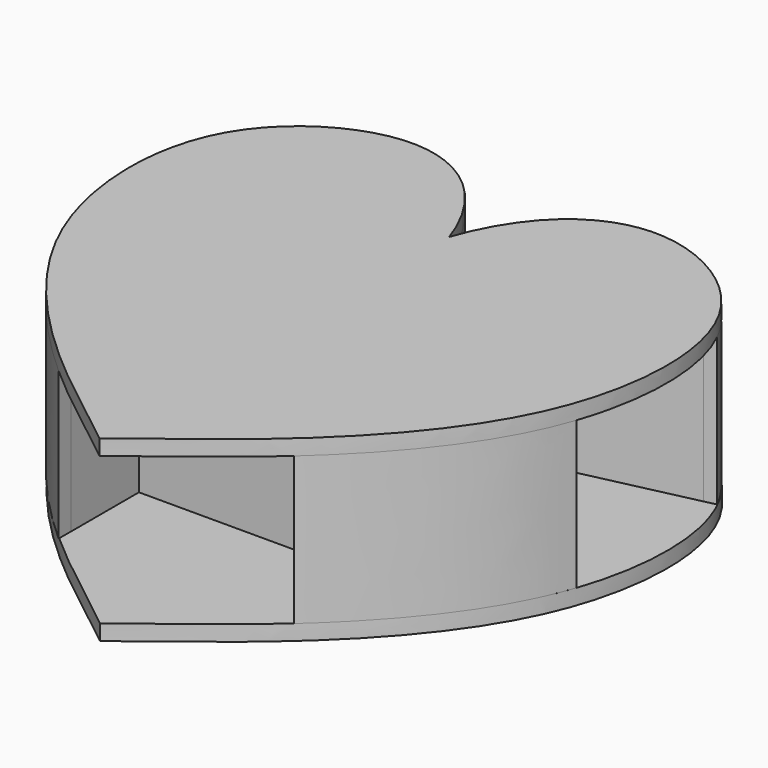
from build123d import *

# Parameters (mm, degrees)
F2_DEPTH = 4
F3_DEPTH = 38
F5_DEPTH = 4


with BuildPart() as f2:
    # F0 (on Top) → F2 (new body)
    with BuildSketch(Plane.XY):
        with BuildLine():
            add(Edge.make_bspline(
                [(3.5143517643, 10.8369065524), (5.5522846532, 17.0202964238), (13.5635309523, 32.3051806354), (38.0529758977, 42.9182898293), (76.1500396351, 20.8141947476), (73.0025805002, -39.6990670077), (29.4912941702, -82.5722333451), (15.9784645563, -91.4802309528), (3.4199764202, -101.6168494477)],
                knots=[0.0076976703, 0.0076976703, 0.0076976703, 0.0076976703, 0.131813136, 0.2661763282, 0.4305411385, 0.6322498153, 0.8376192768, 0.9988747062, 0.9988747062, 0.9988747062, 0.9988747062], degree=3))
            add(Edge.make_bspline(
                [(3.5143517643, 10.8369065524), (1.4767227153, 17.0191988842), (-6.5350491987, 32.3060784633), (-31.0244195059, 42.9171319232), (-67.2133981013, 21.9251415174), (-67.2434681856, -12.7623719687), (-61.6206986806, -29.3254648223)],
                knots=[0.0076974584, 0.0076974584, 0.0076974584, 0.0076974584, 0.1317842693, 0.2661180362, 0.430446851, 0.6070681111, 0.6070681111, 0.6070681111, 0.6070681111], degree=3))
            add(Edge.make_bspline(
                [(-61.6206986806, -29.3254648223), (-60.8234425431, -31.6739565081), (-52.4468997731, -53.0172398251), (-22.4898889785, -82.4508519177), (-9.0233623554, -91.5794035072), (3.4199764202, -101.6168494478)],
                knots=[0.6070681111, 0.6070681111, 0.6070681111, 0.6070681111, 0.6321113542, 0.8374358402, 0.9980646384, 0.9980646384, 0.9980646384, 0.9980646384], degree=3))
        make_face()
    extrude(amount=-F2_DEPTH)

    # F1 (on Top) → F3 (join)
    with BuildSketch(Plane.XY):
        with BuildLine():
            Line((3.4561579753, 4.9706855789), (3.4561579753, 10.7144238582))
            add(Edge.make_bspline(
                [(3.4561579753, 10.7144238582), (1.4185289263, 16.8967161901), (-6.5932429877, 32.1835957691), (-31.0826132949, 42.7946492291), (-54.2586567025, 29.3510180535), (-60.7562355129, 16.9580322491), (-60.9674526745, 16.5360577067)],
                knots=[0.0076974584, 0.0076974584, 0.0076974584, 0.0076974584, 0.1317842693, 0.2661180362, 0.430446851, 0.4361642042, 0.4361642042, 0.4361642042, 0.4361642042], degree=3))
            Line((-60.9674526745, 16.5360577067), (-58.0076894224, 15.867680681))
            add(Edge.make_bspline(
                [(0.6479399733, 9.7061794304), (0.6046874636, 9.8469388096), (0.2425584, 11.0072172518), (-0.7433365613, 13.808672451), (-2.7746951207, 17.9846349652), (-5.4067765074, 22.3254866101), (-8.227454907, 25.8258588748), (-10.9956638863, 28.4577402835), (-13.8782115073, 30.8251417264), (-17.2785962738, 32.9258246007), (-21.0533247221, 34.2378846946), (-24.43835167, 34.841782762), (-27.3674152087, 35.071859033), (-30.1156927854, 34.9731006728), (-32.9581094547, 34.569195533), (-36.2057374717, 33.7631574987), (-40.1912204669, 32.4070557976), (-44.7886427582, 30.1694226431), (-49.0054010757, 27.0313811661), (-52.2822431782, 23.8435342174), (-54.8028625403, 20.9332222243), (-56.6157057067, 18.3435283848), (-57.6173148948, 16.6079375436), (-58.0076894224, 15.867680681)],
                knots=[1.0346969255, 1.0346969255, 1.0346969255, 1.0346969255, 1.4764116286, 4.6804711386, 9.9341891836, 15.3755233357, 19.8806101881, 23.3717041386, 26.8172416279, 31.0622114635, 35.2849692506, 38.7181632425, 41.3564122598, 44.0851089452, 46.950605509, 49.9535976365, 54.1107624907, 59.5638005463, 65.2173136521, 69.7961412229, 73.2590786057, 76.7528432893, 79.2625536342, 79.2625536342, 79.2625536342, 79.2625536342], degree=3))
            Line((0.6479399733, 9.7061794304), (3.4561579753, 4.9706855789))
        make_face()
        with BuildLine():
            add(Edge.make_bspline(
                [(3.4561579753, 10.7144238582), (5.4940908642, 16.8978137296), (13.5053371633, 32.1826979412), (37.9947821087, 42.7958071352), (61.2178280842, 29.3216869282), (67.7148401511, 16.8696405191), (67.9467655848, 16.4017067521)],
                knots=[0.0076976703, 0.0076976703, 0.0076976703, 0.0076976703, 0.131813136, 0.2661763282, 0.4305411385, 0.4368671972, 0.4368671972, 0.4368671972, 0.4368671972], degree=3))
            Line((3.4561579753, 10.7144238582), (3.4561579753, 4.9706855789))
            Line((3.4561579753, 4.9706855789), (6.2643968648, 9.7062252128))
            add(Edge.make_bspline(
                [(6.2643968648, 9.7062252128), (6.3076486729, 9.8469830471), (6.6697378015, 11.0071453652), (7.6553980554, 13.8080845857), (9.6861370738, 17.9831208796), (12.3173154362, 22.3229027777), (15.1369801468, 25.8225494523), (17.9041390829, 28.4542580271), (20.7856825363, 30.8217142867), (24.1848309962, 32.9227969264), (27.9582556119, 34.2357642717), (31.3421507414, 34.8406865104), (34.2701868543, 35.0717329948), (37.0174798546, 34.9740230615), (39.8589626189, 34.5712402368), (43.1056884615, 33.7665178192), (47.0903857798, 32.4121016938), (51.6872631016, 30.1766110563), (55.9041914607, 27.0411903844), (59.1817327794, 23.8559024251), (61.7031894031, 20.9479678244), (63.5524491428, 18.3097055332), (64.5811168155, 16.5190110217), (64.9961785615, 15.7223911545)],
                knots=[1.034745177, 1.034745177, 1.034745177, 1.034745177, 1.4764548012, 4.6801509047, 9.9325497122, 15.3722717754, 19.8761534689, 23.3665208211, 26.8113738629, 31.0555412324, 35.2773405266, 38.7095624039, 41.3469473392, 44.0746442343, 46.9389452952, 49.9408817932, 54.0967228935, 59.5482830735, 65.2003821651, 69.7779367022, 73.2397529952, 76.7321812838, 79.4260754256, 79.4260754256, 79.4260754256, 79.4260754256], degree=3))
            Line((64.9961785615, 15.7223911545), (67.9467655848, 16.4017067521))
        make_face()
        with BuildLine():
            Line((6.2643968648, 9.7062252128), (3.4561579753, 4.9706855789))
            Line((3.4561579753, 4.9706855789), (0.6479399733, 9.7061794304))
            add(Edge.make_bspline(
                [(0.6479399733, 9.7061794304), (0.6046874636, 9.8469388096), (0.2425584, 11.0072172518), (-0.7433365613, 13.808672451), (-2.7746951207, 17.9846349652), (-5.4067765074, 22.3254866101), (-8.227454907, 25.8258588748), (-10.9956638863, 28.4577402835), (-13.8782115073, 30.8251417264), (-17.2785962738, 32.9258246007), (-21.0533247221, 34.2378846946), (-24.43835167, 34.841782762), (-27.3674152087, 35.071859033), (-30.1156927854, 34.9731006728), (-32.9581094547, 34.569195533), (-36.2057374717, 33.7631574987), (-40.1912204669, 32.4070557976), (-44.7886427582, 30.1694226431), (-49.0054010757, 27.0313811661), (-52.2822431782, 23.8435342174), (-54.8028625403, 20.9332222243), (-56.6157057067, 18.3435283848), (-57.6173148948, 16.6079375436), (-58.0076894224, 15.867680681)],
                knots=[1.0346969255, 1.0346969255, 1.0346969255, 1.0346969255, 1.4764116286, 4.6804711386, 9.9341891836, 15.3755233357, 19.8806101881, 23.3717041386, 26.8172416279, 31.0622114635, 35.2849692506, 38.7181632425, 41.3564122598, 44.0851089452, 46.950605509, 49.9535976365, 54.1107624907, 59.5638005463, 65.2173136521, 69.7961412229, 73.2590786057, 76.7528432893, 79.2625536342, 79.2625536342, 79.2625536342, 79.2625536342], degree=3))
            Line((-58.0076894224, 15.867680681), (-57.9465831476, 15.8538815942))
            Line((-57.9465831476, 15.8538815942), (-0.4570892527, 2.9721040336))
            Line((-0.4570892527, 2.9721040336), (-3.7431103507, -11.7157063329))
            Line((-3.7431103507, -11.7157063329), (-10.2986664004, -40.9504371215))
            Line((-10.2986664004, -40.9504371215), (-58.2317647828, -30.201984695))
            Line((-58.2317647828, -30.201984695), (-58.3803942393, -30.1694729501))
            add(Edge.make_bspline(
                [(-58.3803942393, -30.1694729501), (-58.1555596349, -30.7636155671), (-57.1914047793, -33.2104050549), (-55.2539965122, -37.4204653201), (-52.261503605, -43.2065561699), (-48.2577140945, -49.5745432001), (-43.1622417941, -56.2991762185), (-37.7802365002, -62.5431818573), (-32.897833219, -67.5664981209), (-29.1434884385, -71.1923826424), (-27.0245490324, -73.1666145526), (-26.1856401319, -73.9345530884)],
                knots=[126.5893078984, 126.5893078984, 126.5893078984, 126.5893078984, 128.4943272239, 134.4758365242, 140.4840464521, 148.0263281727, 157.0085926933, 165.7708543176, 172.7401643843, 178.0161441156, 181.428082058, 181.428082058, 181.428082058, 181.428082058], degree=3))
            Line((-26.1856401319, -73.9345530884), (-26.1855794561, -73.9194649769))
            Line((-26.1855794561, -73.9194649769), (-26.1855794561, -52.1151364364))
            Line((-26.1855794561, -52.1151364364), (3.8144205439, -52.1151364364))
            Line((3.8144205439, -52.1151364364), (33.8144205439, -52.1151364364))
            Line((33.8144205439, -52.1151364364), (33.8144205439, -73.2800545906))
            Line((33.8144205439, -73.2800545906), (33.8145978261, -73.295787078))
            add(Edge.make_bspline(
                [(65.2226804963, -30.3470502278), (65.0237913966, -30.8686445443), (64.0856409406, -33.2436350348), (62.183747075, -37.3870630535), (59.1957142226, -43.1787098395), (55.197398604, -49.5539356548), (50.1072963279, -56.2861455606), (44.7295313025, -62.5353271551), (39.8489959503, -67.5590883153), (36.3155537504, -70.9682702153), (34.4244042671, -72.7336646435), (33.8145978261, -73.295787078)],
                knots=[126.7787238633, 126.7787238633, 126.7787238633, 126.7787238633, 128.4527743373, 134.4366412672, 140.4475244108, 147.9934656014, 156.9790826267, 165.7426161188, 172.7105318281, 177.9834554998, 180.4715207481, 180.4715207481, 180.4715207481, 180.4715207481], degree=3))
            Line((65.2226804963, -30.3470502278), (65.0778019164, -30.3775195831))
            Line((65.0778019164, -30.3775195831), (17.9275074882, -40.9504371215))
            Line((17.9275074882, -40.9504371215), (11.3719514384, -11.7157063329))
            Line((11.3719514384, -11.7157063329), (8.0859303405, 2.9721040336))
            Line((8.0859303405, 2.9721040336), (64.9340126509, 15.7080786559))
            Line((64.9340126509, 15.7080786559), (64.9961785615, 15.7223911545))
            add(Edge.make_bspline(
                [(6.2643968648, 9.7062252128), (6.3076486729, 9.8469830471), (6.6697378015, 11.0071453652), (7.6553980554, 13.8080845857), (9.6861370738, 17.9831208796), (12.3173154362, 22.3229027777), (15.1369801468, 25.8225494523), (17.9041390829, 28.4542580271), (20.7856825363, 30.8217142867), (24.1848309962, 32.9227969264), (27.9582556119, 34.2357642717), (31.3421507414, 34.8406865104), (34.2701868543, 35.0717329948), (37.0174798546, 34.9740230615), (39.8589626189, 34.5712402368), (43.1056884615, 33.7665178192), (47.0903857798, 32.4121016938), (51.6872631016, 30.1766110563), (55.9041914607, 27.0411903844), (59.1817327794, 23.8559024251), (61.7031894031, 20.9479678244), (63.5524491428, 18.3097055332), (64.5811168155, 16.5190110217), (64.9961785615, 15.7223911545)],
                knots=[1.034745177, 1.034745177, 1.034745177, 1.034745177, 1.4764548012, 4.6801509047, 9.9325497122, 15.3722717754, 19.8761534689, 23.3665208211, 26.8113738629, 31.0555412324, 35.2773405266, 38.7095624039, 41.3469473392, 44.0746442343, 46.9389452952, 49.9408817932, 54.0967228935, 59.5482830735, 65.2003821651, 69.7779367022, 73.2397529952, 76.7321812838, 79.4260754256, 79.4260754256, 79.4260754256, 79.4260754256], degree=3))
        make_face()
        with BuildLine():
            Line((-58.3803942393, -30.1694729501), (-61.6788924696, -29.4479475164))
            add(Edge.make_bspline(
                [(-61.6788924696, -29.4479475164), (-60.881636332, -31.7964392023), (-53.0462399942, -51.7608909495), (-37.0967734108, -68.2241063055), (-26.2017837773, -77.9489602814)],
                knots=[0.6070681111, 0.6070681111, 0.6070681111, 0.6070681111, 0.6321113542, 0.8225534862, 0.8225534862, 0.8225534862, 0.8225534862], degree=3))
            Line((-26.2017837773, -77.9489602814), (-26.1856401319, -73.9345530884))
            add(Edge.make_bspline(
                [(-58.3803942393, -30.1694729501), (-58.1555596349, -30.7636155671), (-57.1914047793, -33.2104050549), (-55.2539965122, -37.4204653201), (-52.261503605, -43.2065561699), (-48.2577140945, -49.5745432001), (-43.1622417941, -56.2991762185), (-37.7802365002, -62.5431818573), (-32.897833219, -67.5664981209), (-29.1434884385, -71.1923826424), (-27.0245490324, -73.1666145526), (-26.1856401319, -73.9345530884)],
                knots=[126.5893078984, 126.5893078984, 126.5893078984, 126.5893078984, 128.4943272239, 134.4758365242, 140.4840464521, 148.0263281727, 157.0085926933, 165.7708543176, 172.7401643843, 178.0161441156, 181.428082058, 181.428082058, 181.428082058, 181.428082058], degree=3))
        make_face()
        with BuildLine():
            add(Edge.make_bspline(
                [(68.518907896, -29.6538219824), (67.7390456014, -31.9317266469), (60.0621472753, -51.4272664766), (44.652351305, -67.6078067079), (33.8596555935, -77.2943319762)],
                knots=[0.6079462349, 0.6079462349, 0.6079462349, 0.6079462349, 0.6322498153, 0.8184323199, 0.8184323199, 0.8184323199, 0.8184323199], degree=3))
            Line((68.518907896, -29.6538219824), (65.2226804963, -30.3470502278))
            add(Edge.make_bspline(
                [(65.2226804963, -30.3470502278), (65.0237913966, -30.8686445443), (64.0856409406, -33.2436350348), (62.183747075, -37.3870630535), (59.1957142226, -43.1787098395), (55.197398604, -49.5539356548), (50.1072963279, -56.2861455606), (44.7295313025, -62.5353271551), (39.8489959503, -67.5590883153), (36.3155537504, -70.9682702153), (34.4244042671, -72.7336646435), (33.8145978261, -73.295787078)],
                knots=[126.7787238633, 126.7787238633, 126.7787238633, 126.7787238633, 128.4527743373, 134.4366412672, 140.4475244108, 147.9934656014, 156.9790826267, 165.7426161188, 172.7105318281, 177.9834554998, 180.4715207481, 180.4715207481, 180.4715207481, 180.4715207481], degree=3))
            Line((33.8145978261, -73.295787078), (33.8596555935, -77.2943319762))
        make_face()
    extrude(amount=F3_DEPTH)

    # F4 (on face) → F5 (join)
    with BuildSketch(Plane.XY.offset(38)):
        with BuildLine():
            add(Edge.make_bspline(
                [(3.4561579753, 10.7144238582), (5.4940908642, 16.8978137296), (13.5053371633, 32.1826979412), (37.9947821087, 42.7958071352), (76.0918458462, 20.6917120534), (72.9443867112, -39.8215497018), (29.4331003812, -82.6947160393), (15.9202707673, -91.6027136469), (3.3617826313, -101.7393321419)],
                knots=[0.0076976703, 0.0076976703, 0.0076976703, 0.0076976703, 0.131813136, 0.2661763282, 0.4305411385, 0.6322498153, 0.8376192768, 0.9988747062, 0.9988747062, 0.9988747062, 0.9988747062], degree=3))
            add(Edge.make_bspline(
                [(3.4561579753, 10.7144238582), (1.4185289263, 16.8967161901), (-6.5932429877, 32.1835957691), (-31.0826132949, 42.7946492291), (-67.2715918903, 21.8026588232), (-67.3016619746, -12.8848546628), (-61.6788924696, -29.4479475164)],
                knots=[0.0076974584, 0.0076974584, 0.0076974584, 0.0076974584, 0.1317842693, 0.2661180362, 0.430446851, 0.6070681111, 0.6070681111, 0.6070681111, 0.6070681111], degree=3))
            add(Edge.make_bspline(
                [(-61.6788924696, -29.4479475164), (-60.881636332, -31.7964392023), (-52.5050935621, -53.1397225192), (-22.5480827674, -82.5733346119), (-9.0815561443, -91.7018862014), (3.3617826313, -101.7393321419)],
                knots=[0.6070681111, 0.6070681111, 0.6070681111, 0.6070681111, 0.6321113542, 0.8374358402, 0.9980646384, 0.9980646384, 0.9980646384, 0.9980646384], degree=3))
        make_face()
    extrude(amount=F5_DEPTH)


solid = f2.part
